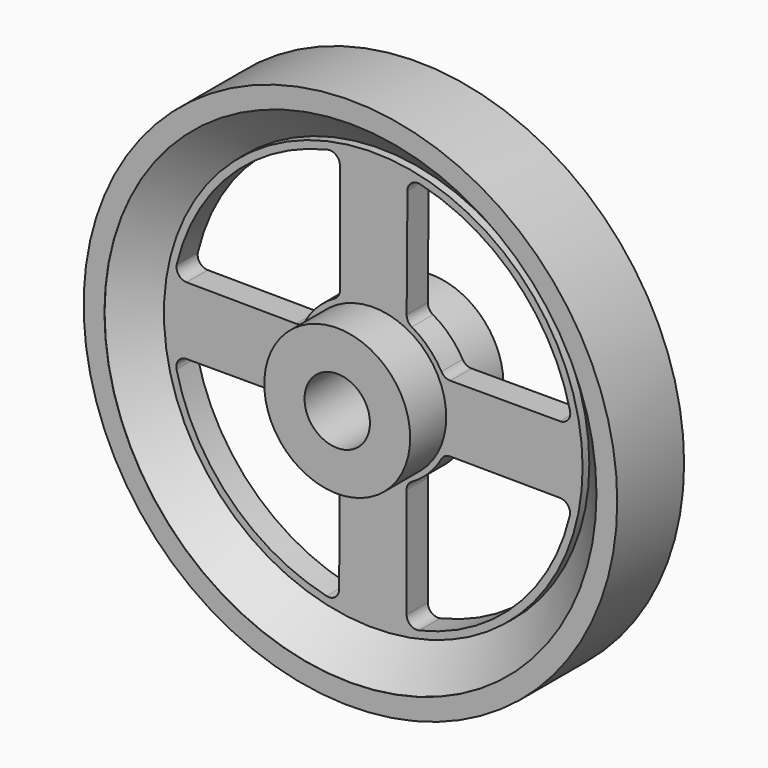
from build123d import *

# Parameters (mm, degrees)
F0_R     = 102.7
F0_R_2   = 35.8
F1_DEPTH = 6.5
F0_R_3   = 16.05
F2_DEPTH = 28.6
F3_R     = 120.7
F3_R_2   = 102.8
F4_DEPTH = 20.5
F3_R_3   = 130.9
F6_DEPTH = 20.5


# Not quite as in the source:
# - a fillet or chamfer that OpenCascade refuses, or shapes differently, is made with other operations: its cross-section is extruded or revolved along the edge and cut away or added


with BuildPart() as f1:
    # F0 (on Front) → F1 (new body, symmetric)
    with BuildSketch(Plane.XZ):
        Circle(F0_R)
        with BuildLine():
            ThreePointArc((-22.9240592059, -96.4121232497), (-70.2337791547, -69.9144210135), (-96.5155963671, -22.4844314559))
            ThreePointArc((-96.5155963671, -22.4844314559), (-95.5621206621, -18.2413151719), (-91.6459900923, -16.35))
            Line((-91.6459900923, -16.35), (-37.7854138524, -16.35))
            ThreePointArc((-37.7854138524, -16.35), (-35.2653332086, -17.031528795), (-33.4322555745, -18.8903225806))
            ThreePointArc((-33.4322555745, -18.8903225806), (-27.1609405883, -27.1448578253), (-18.9101213144, -33.4210609029))
            ThreePointArc((-18.9101213144, -33.4210609029), (-17.0439362056, -35.2698426574), (-16.3725116244, -37.8094941823))
            Line((-16.3725116244, -37.8094941823), (-16.7675816639, -91.5844702575))
            ThreePointArc((-16.7675816639, -91.5844702575), (-18.682125683, -95.4823016351), (-22.9240592059, -96.4121232497))
        make_face(mode=Mode.SUBTRACT)
        Circle(F0_R_2, mode=Mode.SUBTRACT)
        with BuildLine():
            ThreePointArc((16.35, -37.7854138524), (17.031528795, -35.2653332086), (18.8903225806, -33.4322555745))
            ThreePointArc((18.8903225806, -33.4322555745), (27.1448578253, -27.1609405883), (33.4210609029, -18.9101213144))
            ThreePointArc((33.4210609029, -18.9101213144), (35.2698426574, -17.0439362056), (37.8094941823, -16.3725116244))
            Line((37.8094941823, -16.3725116244), (91.5844702575, -16.7675816639))
            ThreePointArc((91.5844702575, -16.7675816639), (95.4823016351, -18.682125683), (96.4121232497, -22.9240592059))
            ThreePointArc((96.4121232497, -22.9240592059), (69.9144210135, -70.2337791547), (22.4844314559, -96.5155963671))
            ThreePointArc((22.4844314559, -96.5155963671), (18.2413151719, -95.5621206621), (16.35, -91.6459900923))
            Line((16.35, -91.6459900923), (16.35, -37.7854138524))
        make_face(mode=Mode.SUBTRACT)
        with BuildLine():
            ThreePointArc((-16.35, 37.7854138524), (-17.031528795, 35.2653332086), (-18.8903225806, 33.4322555745))
            ThreePointArc((-18.8903225806, 33.4322555745), (-27.1448578253, 27.1609405883), (-33.4210609029, 18.9101213144))
            ThreePointArc((-33.4210609029, 18.9101213144), (-35.2698426574, 17.0439362056), (-37.8094941823, 16.3725116244))
            Line((-37.8094941823, 16.3725116244), (-91.5844702575, 16.7675816639))
            ThreePointArc((-91.5844702575, 16.7675816639), (-95.4823016351, 18.682125683), (-96.4121232497, 22.9240592059))
            ThreePointArc((-96.4121232497, 22.9240592059), (-69.9144210135, 70.2337791547), (-22.4844314559, 96.5155963671))
            ThreePointArc((-22.4844314559, 96.5155963671), (-18.2413151719, 95.5621206621), (-16.35, 91.6459900923))
            Line((-16.35, 91.6459900923), (-16.35, 37.7854138524))
        make_face(mode=Mode.SUBTRACT)
        with BuildLine():
            ThreePointArc((37.7854138524, 16.35), (35.2653332086, 17.031528795), (33.4322555745, 18.8903225806))
            ThreePointArc((33.4322555745, 18.8903225806), (27.1609405883, 27.1448578253), (18.9101213144, 33.4210609029))
            ThreePointArc((18.9101213144, 33.4210609029), (17.0439362056, 35.2698426574), (16.3725116244, 37.8094941823))
            Line((16.3725116244, 37.8094941823), (16.7675816639, 91.5844702575))
            ThreePointArc((16.7675816639, 91.5844702575), (18.682125683, 95.4823016351), (22.9240592059, 96.4121232497))
            ThreePointArc((22.9240592059, 96.4121232497), (70.2337791547, 69.9144210135), (96.5155963671, 22.4844314559))
            ThreePointArc((96.5155963671, 22.4844314559), (95.5621206621, 18.2413151719), (91.6459900923, 16.35))
            Line((91.6459900923, 16.35), (37.7854138524, 16.35))
        make_face(mode=Mode.SUBTRACT)
    extrude(amount=F1_DEPTH, both=True)

    # F0 (on Front) → F2 (join, symmetric)
    with BuildSketch(Plane.XZ):
        Circle(F0_R_2)
        Circle(F0_R_3, mode=Mode.SUBTRACT)
    extrude(amount=F2_DEPTH, both=True)


with BuildPart() as f4:
    # F3 (on Front) → F4 (new body, symmetric)
    with BuildSketch(Plane.XZ):
        Circle(F3_R)
        Circle(F3_R_2, mode=Mode.SUBTRACT)
    extrude(amount=F4_DEPTH, both=True)

    # F5: chamfer of 18 on 3 edges, made by hand

    # F5_s1 → F5_t2 (revolve, cut)
    with BuildSketch(Plane.XY):
        Polygon((120.8, -20.5), (102.8, -2.5), (102.8, -20.5), align=None)
    revolve(axis=Axis((0, -20.5, 0), (0, -1, 0)), mode=Mode.SUBTRACT)

    # F5_s3 → F5_t4 (revolve, cut)
    with BuildSketch(Plane.XY):
        Polygon((102.8, 2.5), (120.8, 20.5), (102.8, 20.5), align=None)
    revolve(axis=Axis((0, 20.5, 0), (0, -1, 0)), mode=Mode.SUBTRACT)

    # F3 (on Front) → F6 (join, symmetric)
    with BuildSketch(Plane.XZ):
        Circle(F3_R_3)
        Circle(F3_R, mode=Mode.SUBTRACT)
    extrude(amount=F6_DEPTH, both=True)


solid = Compound([f1.part, f4.part])
